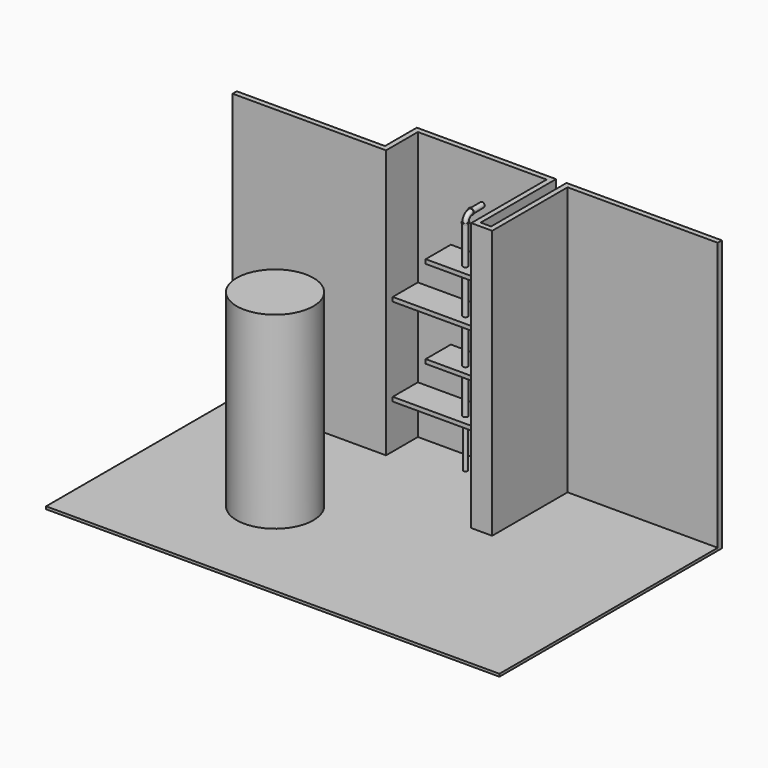
from build123d import *

# Parameters (mm, degrees)
F1_DEPTH  = 25
F3_DEPTH  = 2590
F9_W      = 915
F9_H      = 300
F10_DEPTH = 40
F11_W     = 915
F11_H     = 300
F12_DEPTH = 40
F13_W     = 915
F13_H     = 300
F14_DEPTH = 40
F15_W     = 915
F15_H     = 300
F16_DEPTH = 40
F17_R     = 18.15
F18_DEPTH = 400
F19_R     = 24.15
F20_DEPTH = 1320
F21_R     = 26
F22_DEPTH = 20
F23_R     = 24.15
F24_DEPTH = 400
F25_R     = 34.15
F26_DEPTH = 20
F27_R     = 24.15
F28_DEPTH = 400
F29_R     = 34.15
F30_DEPTH = 20
F31_R     = 24.15
F32_DEPTH = 400
F33_R     = 34.15
F34_DEPTH = 20
F35_R     = 24.15
F36_DEPTH = 400
F37_R     = 29.15
F38_DEPTH = 10
F42_R     = 24.15
F47_R     = 29.15
F48_DEPTH = 5
F49_R     = 24.15
F50_REACH = 252.8226248047
F51_R     = 366.4389442896
F52_DEPTH = 1800
F53_W     = 20
F53_H     = 260
F54_DEPTH = 20


with BuildPart() as f1:
    # F0 (on Top) → F1 (new body)
    with BuildSketch(Plane.XY):
        Polygon((-705.1947621593, 181.9470898961), (-2171.3920796187, 181.9470898961), (-2171.3920796187, -2044.813666757), (2159.594360915, -2044.813666757), (2159.594360915, 561.9470898961), (724.8052378407, 561.9470898961), (724.8052378407, -338.0529101039), (524.8052378407, -338.0529101039), (524.8052378407, 561.9470898961), (-705.1947621593, 561.9470898961), align=None)
    extrude(amount=F1_DEPTH)


with BuildPart() as f3:
    # F2 (on face) → F3 (new body)
    with BuildSketch(Plane(origin=(0, 0, 0), x_dir=(1, 0, 0), z_dir=(0, 0, -1))):
        Polygon((-705.1947621593, -181.9470898961), (-2171.3920796187, -181.9470898961), (-2171.3920796187, -231.9470898961), (-755.1947621593, -231.9470898961), (-755.1947621593, -611.9470898961), (574.8052378407, -611.9470898961), (574.8052378407, 288.0529101039), (674.8052378407, 288.0529101039), (674.8052378407, -611.9470898961), (2159.594360915, -611.9470898961), (2159.594360915, -561.9470898961), (724.8052378407, -561.9470898961), (724.8052378407, 338.0529101039), (524.8052378407, 338.0529101039), (524.8052378407, -561.9470898961), (-705.1947621593, -561.9470898961), align=None)
    extrude(amount=-F3_DEPTH)


with BuildPart() as f10:
    # F9 (on offset) → F10 (new body)
    with BuildSketch(Plane.XY.offset(445)):
        with Locations((-247.6947621593, 411.9470898961)):
            Rectangle(F9_W, F9_H)
    extrude(amount=F10_DEPTH)


with BuildPart() as f12:
    # F11 (on offset) → F12 (new body)
    with BuildSketch(Plane.XY.offset(865)):
        with Locations((67.3052378407, 411.9470898961)):
            Rectangle(F11_W, F11_H)
    extrude(amount=F12_DEPTH)


with BuildPart() as f14:
    # F13 (on offset) → F14 (new body)
    with BuildSketch(Plane.XY.offset(1285)):
        with Locations((-247.6947621593, 411.9470898961)):
            Rectangle(F13_W, F13_H)
    extrude(amount=F14_DEPTH)


with BuildPart() as f16:
    # F15 (on offset) → F16 (new body)
    with BuildSketch(Plane.XY.offset(1705)):
        with Locations((67.3052378407, 411.9470898961)):
            Rectangle(F15_W, F15_H)
    extrude(amount=F16_DEPTH)


with BuildPart() as f18:
    # F17 (on face) → F18 (new body)
    with BuildSketch(Plane.XY.offset(25)):
        with Locations((-90.1947621593, 361.9470898961)):
            Circle(F17_R)
    extrude(amount=F18_DEPTH)

    # F21 (on face) → F22 (join)
    with BuildSketch(Plane.XY.offset(425)):
        with Locations((-90.1947621593, 361.9470898961)):
            Circle(F21_R)
    extrude(amount=F22_DEPTH)

    # F23 (on face) → F24 (join)
    with BuildSketch(Plane.XY.offset(445)):
        with Locations((-90.1947621593, 361.9470898961)):
            Circle(F23_R)
    extrude(amount=F24_DEPTH)

    # F25 (on face) → F26 (join)
    with BuildSketch(Plane.XY.offset(845)):
        with Locations((-90.1947621593, 361.9470898961)):
            Circle(F25_R)
    extrude(amount=F26_DEPTH)

    # F27 (on face) → F28 (join)
    with BuildSketch(Plane.XY.offset(865)):
        with Locations((-90.1947621593, 361.9470898961)):
            Circle(F27_R)
    extrude(amount=F28_DEPTH)

    # F29 (on face) → F30 (join)
    with BuildSketch(Plane.XY.offset(1265)):
        with Locations((-90.1947621593, 361.9470898961)):
            Circle(F29_R)
    extrude(amount=F30_DEPTH)

    # F31 (on face) → F32 (join)
    with BuildSketch(Plane.XY.offset(1285)):
        with Locations((-90.1947621593, 361.9470898961)):
            Circle(F31_R)
    extrude(amount=F32_DEPTH)

    # F33 (on face) → F34 (join)
    with BuildSketch(Plane.XY.offset(1685)):
        with Locations((-90.1947621593, 361.9470898961)):
            Circle(F33_R)
    extrude(amount=F34_DEPTH)

    # F35 (on face) → F36 (join)
    with BuildSketch(Plane.XY.offset(1705)):
        with Locations((-90.1947621593, 361.9470898961)):
            Circle(F35_R)
    extrude(amount=F36_DEPTH)

    # F37 (on face) → F38 (join)
    with BuildSketch(Plane.XY.offset(2105)):
        with Locations((-90.1947621593, 361.9470898961)):
            Circle(F37_R)
    extrude(amount=F38_DEPTH)

    # F46: sweep along a path in F45
    with BuildLine(Plane(origin=(-90.1947621593, 0, 0), x_dir=(0, -1, 0), z_dir=(-1, 0, 0))) as f46_path:
        ThreePointArc((-361.9470898961, 2115), (-381.8016351531, 2159.12457081), (-426.9470898961, 2176.5334373028))
    # F42 (on face) → F46 (sweep)
    with BuildSketch(Plane.XY.offset(2115)):
        with Locations((-90.1947621593, 361.9470898961)):
            Circle(F42_R)
    sweep(path=f46_path.line)

    # F47 (on face) → F48 (join)
    with BuildSketch(Plane(origin=(0, 450.7208860992, 4.9343114773), x_dir=(-1, 0, 0), z_dir=(0, 0.9999400804, 0.0109469429))):
        with Locations((90.1947621593, 2171.7292549193)):
            Circle(F47_R)
    extrude(amount=F48_DEPTH)

    f50_end = f3.part.faces().sort_by_distance((-90.1947621593, 561.9470898961, 1295))[0]
    # F49 (on face) → F50 (join, up to a face of F3 that its end follows)
    with BuildSketch(Plane(origin=(0, 455.7205865013, 4.9890461919), x_dir=(-1, 0, 0), z_dir=(0, 0.9999400804, 0.0109469429))):
        with Locations((90.1947621593, 2171.7292549193)):
            Circle(F49_R)
    f50_long = extrude(amount=F50_REACH, mode=Mode.PRIVATE)
    add(split(f50_long, bisect_by=f50_end, keep=Keep.TOP, mode=Mode.PRIVATE))


with BuildPart() as f20_tool:
    # F19 (on face) → F20 (new body)
    with BuildSketch(Plane.XY.offset(1745)):
        with Locations((-90.1947621593, 361.9470898961)):
            Circle(F19_R)
    extrude(amount=-F20_DEPTH)


with BuildPart() as f10_1:
    add(f10.part)

    # F20: cut by f20_tool
    add(f20_tool.part, mode=Mode.SUBTRACT)

    # F53 (on face) → F54 (cut)
    with BuildSketch(Plane(origin=(0, 0, 445), x_dir=(1, 0, 0), z_dir=(0, 0, -1))):
        with Locations((-695.1947621593, -431.9470898961)):
            Rectangle(F53_W, F53_H)
    extrude(amount=-F54_DEPTH, mode=Mode.SUBTRACT)


with BuildPart() as f12_1:
    add(f12.part)

    # F20: cut by f20_tool
    add(f20_tool.part, mode=Mode.SUBTRACT)


with BuildPart() as f14_1:
    add(f14.part)

    # F20: cut by f20_tool
    add(f20_tool.part, mode=Mode.SUBTRACT)


with BuildPart() as f16_1:
    add(f16.part)

    # F20: cut by f20_tool
    add(f20_tool.part, mode=Mode.SUBTRACT)


with BuildPart() as f52:
    # F51 (on face) → F52 (new body)
    with BuildSketch(Plane.XY.offset(25)):
        with Locations((-839.6239876747, -975.0935435295)):
            Circle(F51_R)
    extrude(amount=F52_DEPTH)


solid = Compound([f1.part, f3.part, f18.part, f10_1.part, f12_1.part, f14_1.part, f16_1.part, f52.part])
